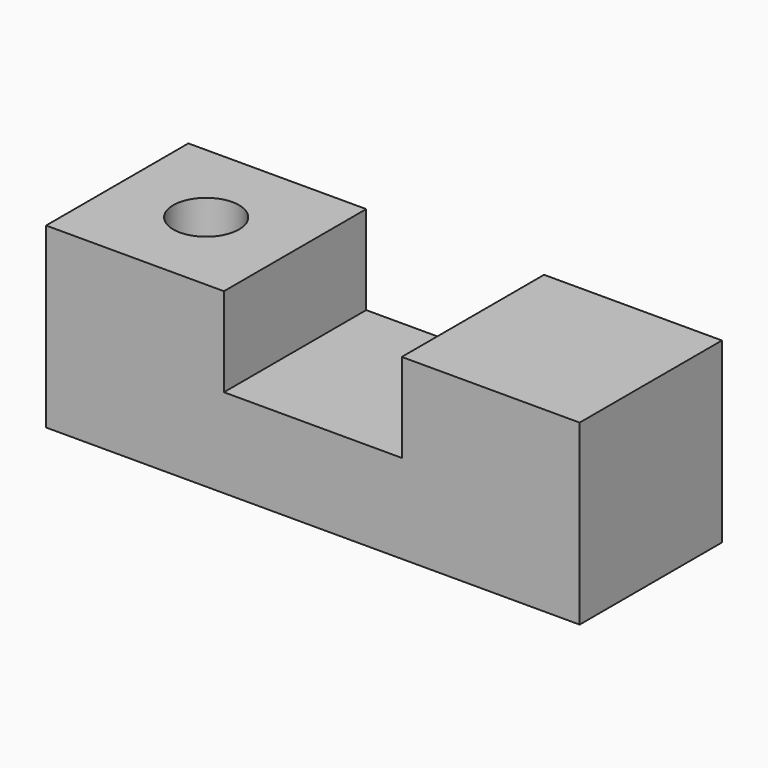
from build123d import *

# Parameters (mm, degrees)
F0_W     = 6.35
F0_H     = 6.35
F0_R     = 1.1751262937
F1_DEPTH = 6.35
F2_DEPTH = 3.175


# Not quite as in the source:
# - a feature names something its author has since deleted; it is built from what else it names


with BuildPart() as f1:
    # F0 (on Top) → F1 (new body)
    with BuildSketch(Plane.XY):
        with Locations((3.175, 3.175)):
            Rectangle(F0_W, F0_H)
        with Locations((3.175, 3.175)):
            Circle(F0_R, mode=Mode.SUBTRACT)
    extrude(amount=F1_DEPTH)



with BuildPart() as f1b:
    # F0 (on Top) → F1, piece 2 (new body)
    with BuildSketch(Plane.XY):
        with Locations((15.875, 3.175)):
            Rectangle(F0_W, F0_H)
    extrude(amount=F1_DEPTH)


with BuildPart() as f1_1:
    add(f1.part)

    add(f1b.part)  # F2 merges F1b
    # F0 (on Top) → F2 (join)
    with BuildSketch(Plane.XY):
        with Locations((9.525, 3.175)):
            Rectangle(F0_W, F0_H)
    extrude(amount=F2_DEPTH)


solid = f1_1.part
